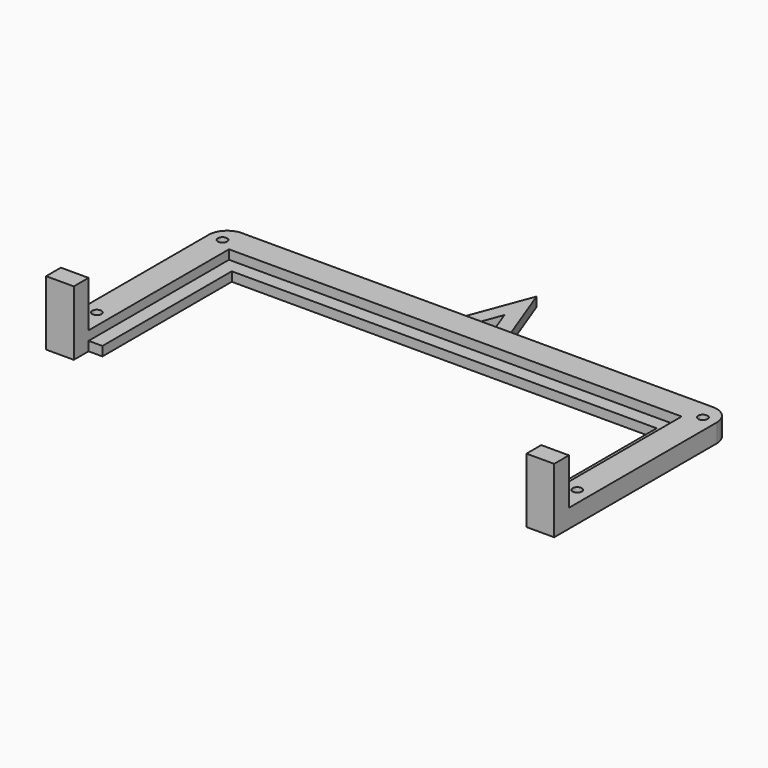
from build123d import *

# Parameters (mm, degrees)
F0_R     = 1.5875
F1_DEPTH = 3.175
F2_DEPTH = 3.175
F3_DEPTH = 19.05


# Not quite as in the source:
# - a feature names something its author has since deleted; it is built from what else it names


with BuildPart() as f1:
    # F0 (on Top) → F1 (new body)
    with BuildSketch(Plane.XY):
        Polygon((-73.025, 26.19375), (73.025, 26.19375), (73.025, -26.19375), (73.025, -29.36875), (77.7875, -29.36875), (77.7875, -26.19375), (77.7875, 30.95625), (-77.7875, 30.95625), (-77.7875, -26.19375), (-77.7875, -29.36875), (-73.025, -29.36875), (-73.025, -26.19375), align=None)
        with BuildLine():
            Line((77.7875, -26.19375), (77.7875, -29.36875))
            Line((77.7875, -29.36875), (87.3125, -29.36875))
            Line((87.3125, -29.36875), (87.3125, -26.19375))
            Line((87.3125, -26.19375), (87.3125, 34.1312500767))
            ThreePointArc((87.3125, 34.1312500767), (85.452628083, 38.621378083), (80.9625000767, 40.48125))
            Line((80.9625000767, 40.48125), (9.525, 40.48125))
            Line((9.525, 40.48125), (7.9375, 40.48125))
            Line((7.9375, 40.48125), (4.3422256552, 40.48125))
            Line((4.3422256552, 40.48125), (-1.5875, 40.48125))
            Line((-1.5875, 40.48125), (-4.3422256552, 40.48125))
            Line((-4.3422256552, 40.48125), (-9.525, 40.48125))
            Line((-9.525, 40.48125), (-80.9625000767, 40.48125))
            ThreePointArc((-80.9625000767, 40.48125), (-85.452628083, 38.621378083), (-87.3125, 34.1312500767))
            Line((-87.3125, 34.1312500767), (-87.3125, -26.19375))
            Line((-87.3125, -26.19375), (-87.3125, -29.36875))
            Line((-87.3125, -29.36875), (-77.7875, -29.36875))
            Line((-77.7875, -29.36875), (-77.7875, -26.19375))
            Line((-77.7875, -26.19375), (-77.7875, 30.95625))
            Line((-77.7875, 30.95625), (77.7875, 30.95625))
            Line((77.7875, 30.95625), (77.7875, -26.19375))
        make_face()
        with Locations((-82.55, -19.84375)):
            Circle(F0_R, mode=Mode.SUBTRACT)
        with Locations((82.55, -19.84375)):
            Circle(F0_R, mode=Mode.SUBTRACT)
        with Locations((-82.55, 34.13125)):
            Circle(F0_R, mode=Mode.SUBTRACT)
        with Locations((82.55, 34.13125)):
            Circle(F0_R, mode=Mode.SUBTRACT)
        Polygon((-77.7875, -32.54375), (-77.7875, -29.36875), (-87.3125, -29.36875), (-87.3125, -32.54375), (-87.3125, -35.71875), (-77.7875, -35.71875), align=None)
        Polygon((87.3125, -29.36875), (77.7875, -29.36875), (77.7875, -32.54375), (77.7875, -35.71875), (87.3125, -35.71875), (87.3125, -32.54375), align=None)
        Polygon((7.9375, 40.48125), (9.525, 40.48125), (0, 65.88125), (-9.525, 40.48125), (-4.3422256552, 40.48125), (0, 52.0605184138), (4.3422256552, 40.48125), align=None)
    extrude(amount=-F1_DEPTH)

    # F0 (on Top) → F2 (join)
    with BuildSketch(Plane.XY):
        with BuildLine():
            Line((77.7875, -26.19375), (77.7875, -29.36875))
            Line((77.7875, -29.36875), (87.3125, -29.36875))
            Line((87.3125, -29.36875), (87.3125, -26.19375))
            Line((87.3125, -26.19375), (87.3125, 34.1312500767))
            ThreePointArc((87.3125, 34.1312500767), (85.452628083, 38.621378083), (80.9625000767, 40.48125))
            Line((80.9625000767, 40.48125), (9.525, 40.48125))
            Line((9.525, 40.48125), (7.9375, 40.48125))
            Line((7.9375, 40.48125), (4.3422256552, 40.48125))
            Line((4.3422256552, 40.48125), (-1.5875, 40.48125))
            Line((-1.5875, 40.48125), (-4.3422256552, 40.48125))
            Line((-4.3422256552, 40.48125), (-9.525, 40.48125))
            Line((-9.525, 40.48125), (-80.9625000767, 40.48125))
            ThreePointArc((-80.9625000767, 40.48125), (-85.452628083, 38.621378083), (-87.3125, 34.1312500767))
            Line((-87.3125, 34.1312500767), (-87.3125, -26.19375))
            Line((-87.3125, -26.19375), (-87.3125, -29.36875))
            Line((-87.3125, -29.36875), (-77.7875, -29.36875))
            Line((-77.7875, -29.36875), (-77.7875, -26.19375))
            Line((-77.7875, -26.19375), (-77.7875, 30.95625))
            Line((-77.7875, 30.95625), (77.7875, 30.95625))
            Line((77.7875, 30.95625), (77.7875, -26.19375))
        make_face()
        with Locations((-82.55, -19.84375)):
            Circle(F0_R, mode=Mode.SUBTRACT)
        with Locations((82.55, -19.84375)):
            Circle(F0_R, mode=Mode.SUBTRACT)
        with Locations((-82.55, 34.13125)):
            Circle(F0_R, mode=Mode.SUBTRACT)
        with Locations((82.55, 34.13125)):
            Circle(F0_R, mode=Mode.SUBTRACT)
    extrude(amount=F2_DEPTH)

    # F0 (on Top) → F3 (join)
    with BuildSketch(Plane.XY):
        Polygon((87.3125, -29.36875), (77.7875, -29.36875), (77.7875, -32.54375), (77.7875, -35.71875), (87.3125, -35.71875), (87.3125, -32.54375), align=None)
        Polygon((-77.7875, -32.54375), (-77.7875, -29.36875), (-87.3125, -29.36875), (-87.3125, -32.54375), (-87.3125, -35.71875), (-77.7875, -35.71875), align=None)
    extrude(amount=F3_DEPTH)


solid = f1.part
